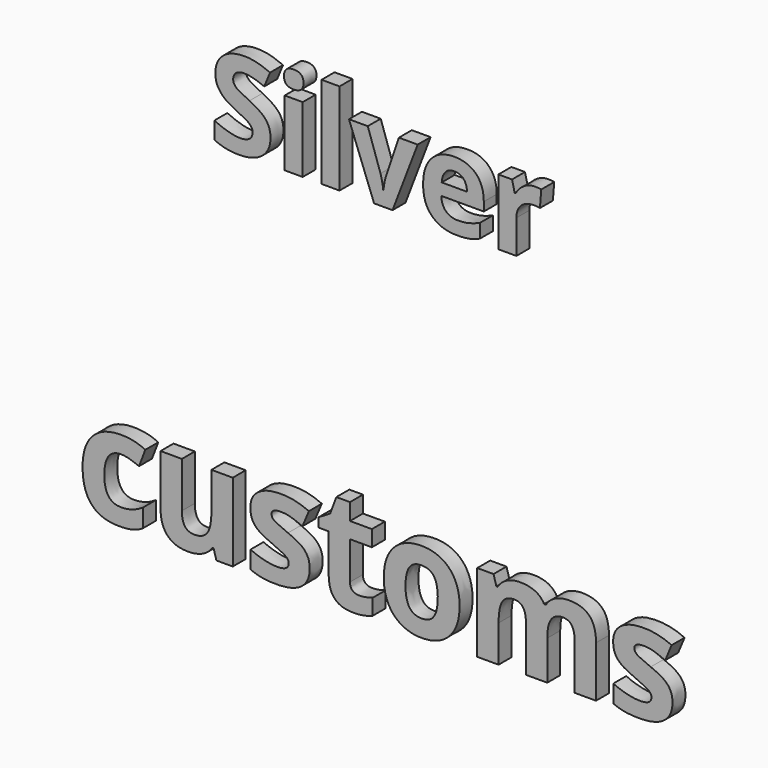
from build123d import *

# Parameters (mm, degrees)
F0_TEXT_SIZE   = 30.7566486299
F0_TEXT_SIZE_2 = 36.4961516526
F1_DEPTH       = 4.1253007948


# Not quite as in the source:
# - Text() gives the source's letters only with a copy of the font that has no kerning and outlines rounded to 1/6400 em; it was checked with that copy


with BuildPart() as f1:
    # F0 (on Front) → F1 (new body)
    with BuildSketch(Plane.XZ):
        with Locations((-43.3476516628, 37.1501147747)):
            Text('Silver', F0_TEXT_SIZE, font='Open Sans', font_style=FontStyle.BOLD, text_align=(TextAlign.LEFT, TextAlign.BOTTOM))
        with Locations((-77.1437405557, -56.0074299574)):
            Text('customs', F0_TEXT_SIZE_2, font='Open Sans', font_style=FontStyle.BOLD, text_align=(TextAlign.LEFT, TextAlign.BOTTOM))
    extrude(amount=F1_DEPTH)


solid = f1.part
